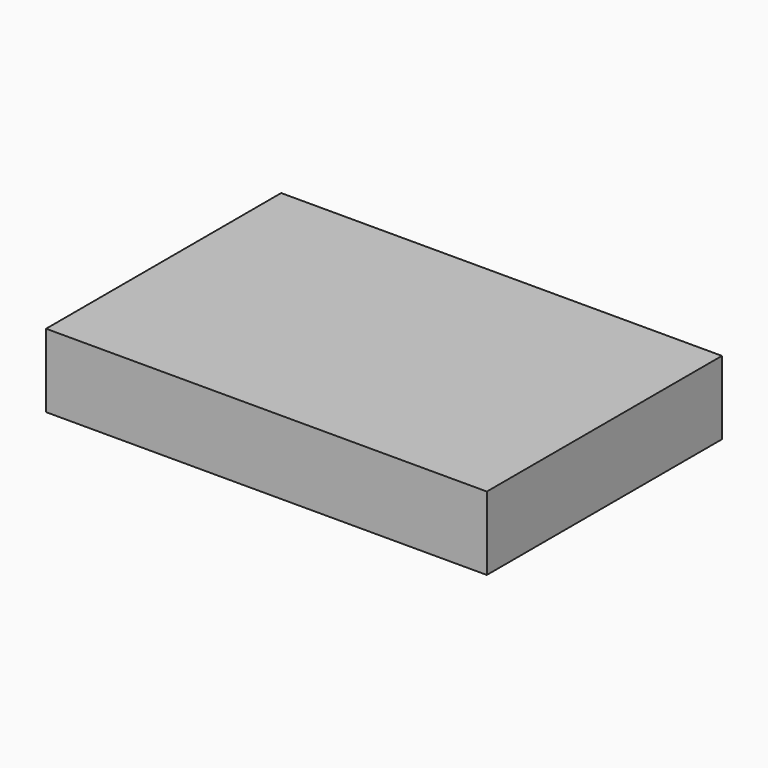
from build123d import *

# Parameters (mm, degrees)
F0_W     = 152.4
F0_H     = 101.6
F1_DEPTH = 25.4


# Not quite as in the source:
# - a feature of the source that left no trace in its solid (it failed there, or was rolled back) is left out


with BuildPart() as f1:
    # F0 (on Top) → F1 (new body)
    with BuildSketch(Plane.XY):
        Rectangle(F0_W, F0_H)
    extrude(amount=F1_DEPTH)


solid = f1.part
